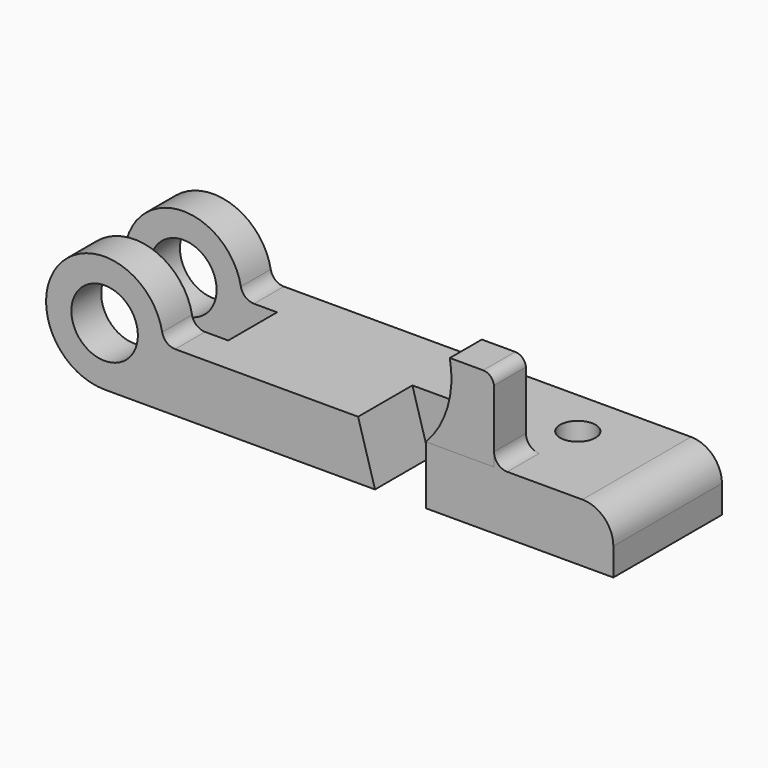
from build123d import *

# Parameters (mm, degrees)
F0_R          = 12.7
F4_DEPTH      = 25.908
F5_DEPTH      = 14.732
F5_DEPTH_BACK = 0.5334
F6_DEPTH      = 51.816
F7_R          = 6.7567647924
F8_DEPTH      = 76.454
F10_DEPTH     = 115.57
F11_R         = 5.08


with BuildPart() as f4:
    # F0 (on Front) → F4 (new body, symmetric)
    with BuildSketch(Plane.XZ):
        with BuildLine():
            Line((182.4113020967, 0), (22.352, 0))
            ThreePointArc((22.352, 0), (-15.8052507731, 15.8052507731), (0, -22.352))
            Line((0, -22.352), (194.2084, -22.352))
            Line((194.2084, -22.352), (194.2084, -11.7970979033))
            ThreePointArc((194.2084, -11.7970979033), (190.7531100225, -3.4552899775), (182.4113020967, 0))
        make_face()
        Circle(F0_R, mode=Mode.SUBTRACT)
    extrude(amount=F4_DEPTH, both=True)

    # F3 (on offset) → F5 (join, two sides)
    with BuildSketch(Plane.XZ.offset(25.4)) as f5_sk:
        with BuildLine():
            ThreePointArc((131.8115741014, 31.148834154), (130.990690219, 14.4909643817), (122.7341517806, 0))
            Line((122.7341517806, 0), (148.645862937, 0))
            Line((148.645862937, 0), (148.645862937, 27.3769088089))
            ThreePointArc((148.645862937, 27.3769088089), (147.3251483028, 30.062921432), (144.5359289646, 31.148834154))
            Line((144.5359289646, 31.148834154), (131.8115741014, 31.148834154))
        make_face()
    extrude(amount=-F5_DEPTH)
    extrude(f5_sk.sketch, amount=F5_DEPTH_BACK)

    # F1 (on Top) → F6 (cut, symmetric)
    with BuildSketch(Plane.XY):
        Polygon((-22.3446302116, 11.6586), (-22.3446302116, 0), (-22.3446302116, -11.6587262601), (35.7894971967, -11.6587262601), (35.7894971967, 11.6586), align=None)
    extrude(amount=F6_DEPTH, both=True, mode=Mode.SUBTRACT)

    # F7 (on Top) → F8 (cut)
    with BuildSketch(Plane.XY):
        with Locations((153.7918448448, 7.6698409393)):
            Circle(F7_R)
    extrude(amount=-F8_DEPTH, mode=Mode.SUBTRACT)

    # F9 (on Front) → F10 (cut)
    with BuildSketch(Plane.XZ):
        Polygon((122.7312460542, -22.4210973829), (122.7312460542, 0), (96.7673584819, 0), (103.2488569617, -22.4210973829), align=None)
    extrude(amount=F10_DEPTH, mode=Mode.SUBTRACT)

    # F11
    f11_edges = [f4.edges().sort_by_distance(p)[0] for p in [
        (22.352, -18.783363, 0),
        (22.352, 18.7833, 0),
        (148.645863, -18.288, 0),
    ]]
    fillet(f11_edges, radius=F11_R)


solid = f4.part
